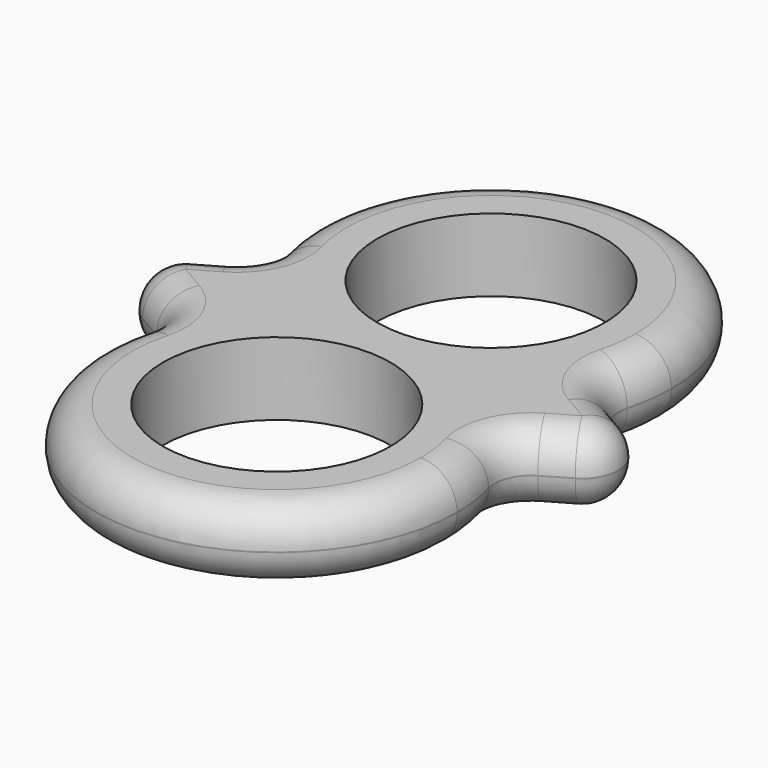
from build123d import *

# Parameters (mm, degrees)
F1_DEPTH = 7.075
F3_DEPTH = 7.075
F4_D     = 22.075
F4_DEPTH = 35.375
F4_TIP   = 6.6319990825
F5_F1_R  = 3.5
F5_F2_R  = 3.5
F5_F3_R  = 3.5


# Not quite as in the source:
# - a pattern or mirror of a feature is missing from the dataset's text; its kind, count and spacing are read off the source's solid


with BuildPart() as f1:
    # F0 (on Top) → F1 (new body)
    with BuildSketch(Plane.XY):
        with BuildLine():
            ThreePointArc((11.7153745139, 0), (15.9885748895, 5.8855447852), (17.5, 13))
            ThreePointArc((17.5, 13), (-7.1144552148, 28.9885748895), (-11.7153745139, 0))
            ThreePointArc((-11.7153745139, 0), (0, 4.5), (11.7153745139, 0))
        make_face()
        with BuildLine():
            ThreePointArc((11.7153745139, 0), (0, -4.5), (-11.7153745139, 0))
            ThreePointArc((-11.7153745139, 0), (-7.1144552148, -28.9885748895), (17.5, -13))
            ThreePointArc((17.5, -13), (15.9885748895, -5.8855447852), (11.7153745139, 0))
        make_face()
        with BuildLine():
            ThreePointArc((11.7153745139, 0), (0, 4.5), (-11.7153745139, 0))
            ThreePointArc((-11.7153745139, 0), (0, -4.5), (11.7153745139, 0))
        make_face()
    extrude(amount=F1_DEPTH)

    # F2 (on Top) → F3 (join)
    with BuildSketch(Plane.XY):
        Polygon((26.25, 0), (0, 15.1554445662), (0, -15.1554445662), align=None)
    f3 = extrude(amount=F3_DEPTH)

    # F3_copies: F3 across plane
    add(f3.mirror(Plane(origin=(0, 0, 0), x_dir=(0, 0, -1), z_dir=(-1, 0, 0))))

    # F4
    with Locations(Plane(origin=(0, 0, 0), x_dir=(1, 0, 0), z_dir=(0, 0, -1))):
        with Locations((0, -13), (0, 13)):
            Hole(F4_D / 2, depth=F4_DEPTH)
            with Locations((0, 0, -(F4_DEPTH + F4_TIP / 2))):  # 118° drill point
                Cone(0, F4_D / 2, F4_TIP, mode=Mode.SUBTRACT)

    # F5: fillet of radius 3.5 on 14 edges, made by hand

    # F5_f1
    f5_f1_edges = [f1.edges().sort_by_distance(p)[0] for p in [
        (16.0023148685, -5.9165037693, 3.5375),
        (-16.0023148685, 5.9165037693, 3.5375),
        (16.0023148685, 5.9165037693, 3.5375),
        (-16.0023148685, -5.9165037693, 3.5375),
    ]]
    fillet(f5_f1_edges, radius=F5_F1_R)

    # F5_f2
    f5_f2_edges = [f1.edges().sort_by_distance(p)[0] for p in [
        (26.25, 0, 3.5375),
        (-26.25, 0, 3.5375),
    ]]
    fillet(f5_f2_edges, radius=F5_F2_R)

    # F5_f3
    f5_f3_edges = [f1.edges().sort_by_distance(p)[0] for p in [
        (19.7579861931, -3.748165919, 0),
        (19.7579861931, -3.748165919, 7.075),
        (0, 30.5, 0),
        (0, 30.5, 7.075),
        (0, -30.5, 0),
        (0, -30.5, 7.075),
        (19.7579861931, 3.748165919, 0),
        (19.7579861931, 3.748165919, 7.075),
        (22.75, 0, 7.075),
        (17.03013711, 6.1624015307, 7.075),
        (22.75, 0, 0),
        (17.03013711, 6.1624015307, 0),
        (-17.03013711, -6.1624015307, 7.075),
        (17.03013711, -6.1624015307, 7.075),
        (-17.03013711, -6.1624015307, 0),
        (17.03013711, -6.1624015307, 0),
        (-17.03013711, 6.1624015307, 7.075),
        (-17.03013711, 6.1624015307, 0),
    ]]
    fillet(f5_f3_edges, radius=F5_F3_R)


solid = f1.part
